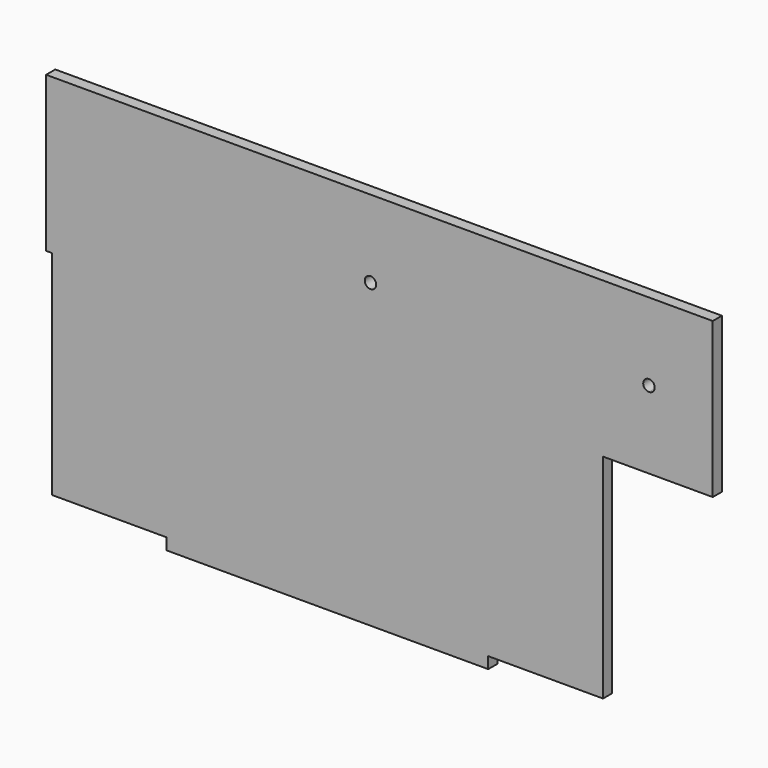
from build123d import *

# Parameters (mm, degrees)
F0_W     = 1
F0_H     = 5
F1_DEPTH = 2
F2_DEPTH = 2


# Not quite as in the source:
# - a feature names something its author has since deleted; it is built from what else it names


with BuildPart() as f1:
    # F0 (on Front) → F1 (new body)
    with BuildSketch(Plane.XZ):
        Polygon((-11.0105917081, 20.8667229116), (-10.0105917081, 20.8667229116), (-10.0105917081, 15.8667229116), (-10.0105917081, -14.7727085277), (-10.0105917081, -21.2332770884), (9.9894082919, -21.2332770884), (9.9894082919, -23.2332770884), (37.9894082919, -23.2332770884), (65.9894082919, -23.2332770884), (65.9894082919, -21.2332770884), (85.9894082919, -21.2332770884), (85.9894082919, -14.7727085277), (85.9894082919, 15.8667229116), (98.9894082919, 15.8667229116), (103.9894082919, 15.8667229116), (105.0934082919, 15.8667229116), (105.0934082919, 42.8667229116), (103.9894082919, 42.8667229116), (98.9894082919, 42.8667229116), (93.9894082919, 42.8667229116), (37.9894082919, 42.8667229116), (-10.0105917081, 42.8667229116), (-11.0105917081, 42.8667229116), align=None)
        with BuildLine():
            ThreePointArc((46.4894082919, 29.3667229116), (45.4894082919, 28.3667229116), (44.4894082919, 29.3667229116))
            ThreePointArc((44.4894082919, 29.3667229116), (45.4894082919, 30.3667229116), (46.4894082919, 29.3667229116))
        make_face(mode=Mode.SUBTRACT)
        with BuildLine():
            ThreePointArc((93.9894082919, 28.3667229116), (93.2823015107, 30.0738296928), (94.9894082919, 29.3667229116))
            ThreePointArc((94.9894082919, 29.3667229116), (94.6965150731, 28.6596161304), (93.9894082919, 28.3667229116))
        make_face(mode=Mode.SUBTRACT)
        with Locations((-10.5105917081, 18.3667229116)):
            Rectangle(F0_W, F0_H)
    extrude(amount=F1_DEPTH)

    # F0 (on Front) → F2 (join)
    with BuildSketch(Plane.XZ):
        Polygon((-11.0105917081, 20.8667229116), (-10.0105917081, 20.8667229116), (-10.0105917081, 15.8667229116), (-10.0105917081, -14.7727085277), (-10.0105917081, -21.2332770884), (9.9894082919, -21.2332770884), (9.9894082919, -23.2332770884), (37.9894082919, -23.2332770884), (65.9894082919, -23.2332770884), (65.9894082919, -21.2332770884), (85.9894082919, -21.2332770884), (85.9894082919, -14.7727085277), (85.9894082919, 15.8667229116), (98.9894082919, 15.8667229116), (103.9894082919, 15.8667229116), (105.0934082919, 15.8667229116), (105.0934082919, 42.8667229116), (103.9894082919, 42.8667229116), (98.9894082919, 42.8667229116), (93.9894082919, 42.8667229116), (37.9894082919, 42.8667229116), (-10.0105917081, 42.8667229116), (-11.0105917081, 42.8667229116), align=None)
        with BuildLine():
            ThreePointArc((46.4894082919, 29.3667229116), (45.4894082919, 28.3667229116), (44.4894082919, 29.3667229116))
            ThreePointArc((44.4894082919, 29.3667229116), (45.4894082919, 30.3667229116), (46.4894082919, 29.3667229116))
        make_face(mode=Mode.SUBTRACT)
        with BuildLine():
            ThreePointArc((93.9894082919, 28.3667229116), (93.2823015107, 30.0738296928), (94.9894082919, 29.3667229116))
            ThreePointArc((94.9894082919, 29.3667229116), (94.6965150731, 28.6596161304), (93.9894082919, 28.3667229116))
        make_face(mode=Mode.SUBTRACT)
    extrude(amount=F2_DEPTH)


solid = f1.part
